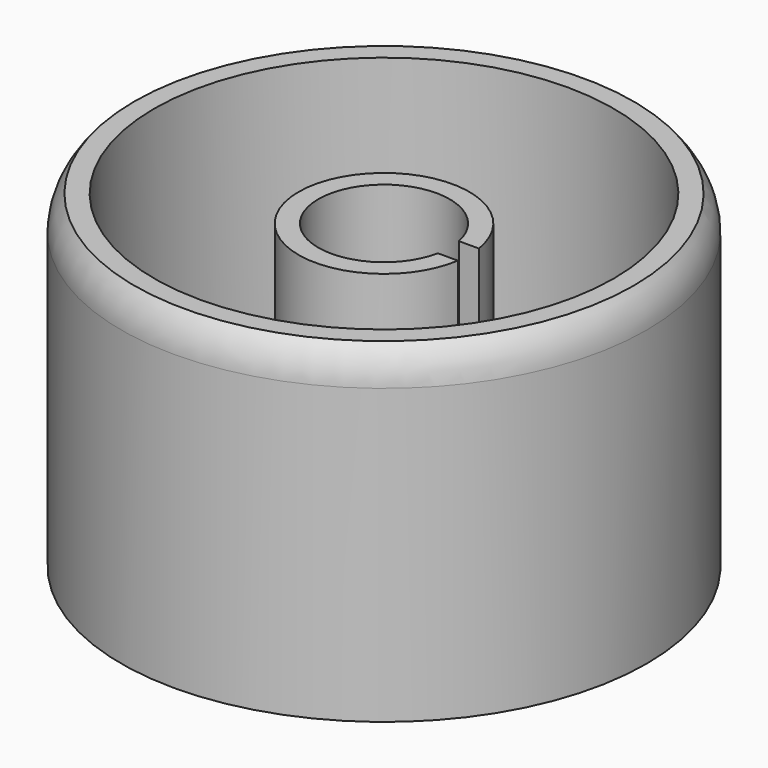
from build123d import *

# Parameters (mm, degrees)
F0_R      = 50.8
F1_DEPTH  = 63.5
F2_R      = 44.45
F3_DEPTH  = 55.88
F4_R      = 44.45
F5_DEPTH  = 2.54
F6_SIZE   = 2.54
F8_R      = 16.51
F8_R_2    = 12.7
F9_DEPTH  = 50.8
F11_DEPTH = 44.45


# Not quite as in the source:
# - a fillet or chamfer that OpenCascade refuses, or shapes differently, is made with other operations: its cross-section is extruded or revolved along the edge and cut away or added


with BuildPart() as f1:
    # F0 (on Top) → F1 (new body)
    with BuildSketch(Plane.XY):
        Circle(F0_R)
    extrude(amount=F1_DEPTH)

    # F2 (on face) → F3 (cut)
    with BuildSketch(Plane.XY.offset(63.5)):
        Circle(F2_R)
    extrude(amount=-F3_DEPTH, mode=Mode.SUBTRACT)

    # F4 (on face) → F5 (cut)
    with BuildSketch(Plane(origin=(0, 0, 0), x_dir=(1, 0, 0), z_dir=(0, 0, -1))):
        Circle(F4_R)
    extrude(amount=-F5_DEPTH, mode=Mode.SUBTRACT)

    # F6
    f6_edges = [f1.edges().sort_by_distance(p)[0] for p in [
        (-50.8, 0, 63.5),
    ]]
    chamfer(f6_edges, length=F6_SIZE)

    # F7: fillet of radius 10.16 on 1 edges, made by hand

    # F7_s1 → F7_t2 (revolve, cut)
    with BuildSketch(Plane.XZ):
        with BuildLine():
            ThreePointArc((50.8, 56.7797916699), (50.1438097624, 60.3718941183), (48.26, 63.5))
            Line((48.26, 63.5), (50.8, 60.96))
            Line((50.8, 60.96), (50.8, 56.7797916699))
        make_face()
    revolve(axis=Axis((0, 0, 60.96), (0, 0, 1)), mode=Mode.SUBTRACT)

    # F8 (on face) → F9 (join)
    with BuildSketch(Plane.XY.offset(7.62)):
        Circle(F8_R)
        Circle(F8_R_2, mode=Mode.SUBTRACT)
    extrude(amount=F9_DEPTH)

    # F10 (on face) → F11 (cut)
    with BuildSketch(Plane.XY.offset(58.42)):
        with BuildLine():
            ThreePointArc((12.4434078933, 2.54), (12.6356891432, 1.2764638175), (12.7, 0))
            Line((12.7, 0), (14.605, 0))
            Line((14.605, 0), (14.605, 2.54))
            Line((14.605, 2.54), (12.4434078933, 2.54))
        make_face()
        with BuildLine():
            Line((14.605, 2.54), (14.605, 0))
            Line((14.605, 0), (16.51, 0))
            ThreePointArc((16.51, 0), (16.4607879997, 1.2737968559), (16.3134453749, 2.54))
            Line((16.3134453749, 2.54), (14.605, 2.54))
        make_face()
        with BuildLine():
            Line((16.51, 0), (14.605, 0))
            Line((14.605, 0), (14.605, -2.54))
            Line((14.605, -2.54), (16.3134453749, -2.54))
            ThreePointArc((16.3134453749, -2.54), (16.4607879997, -1.2737968559), (16.51, 0))
        make_face()
        with BuildLine():
            Line((14.605, 0), (12.7, 0))
            ThreePointArc((12.7, 0), (12.6356891432, -1.2764638175), (12.4434078933, -2.54))
            Line((12.4434078933, -2.54), (14.605, -2.54))
            Line((14.605, -2.54), (14.605, 0))
        make_face()
    extrude(amount=-F11_DEPTH, mode=Mode.SUBTRACT)


solid = f1.part
